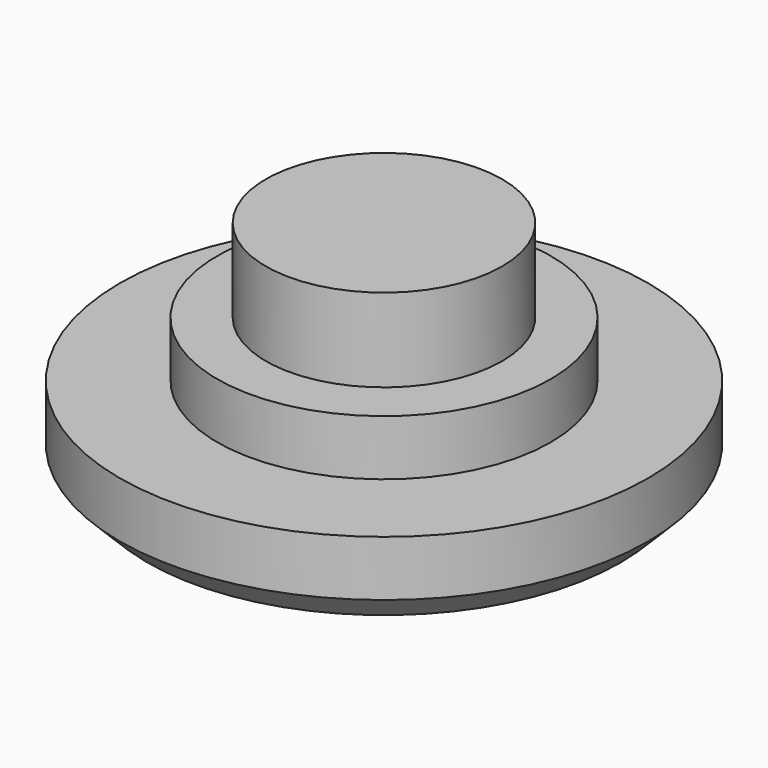
from build123d import *

# Parameters (mm, degrees)
F2_R         = 9.5
F2_R_2       = 6
F3_DEPTH     = 3
F2_R_3       = 4.25
F4_DEPTH     = 5
F5_DEPTH     = 8
F6_SIZE      = 1
F7_TEXT_SIZE = 15.047749256
F8_DEPTH     = 1


# Not quite as in the source:
# - Text() gives the source's letters only with a copy of the font that has no kerning and outlines rounded to 1/6400 em; it was checked with that copy


with BuildPart() as f3:
    # F2 (on Top) → F3 (new body)
    with BuildSketch(Plane.XY):
        Circle(F2_R)
        Circle(F2_R_2, mode=Mode.SUBTRACT)
    extrude(amount=F3_DEPTH)

    # F2 (on Top) → F4 (join)
    with BuildSketch(Plane.XY):
        Circle(F2_R_2)
        Circle(F2_R_3, mode=Mode.SUBTRACT)
    extrude(amount=F4_DEPTH)

    # F2 (on Top) → F5 (join)
    with BuildSketch(Plane.XY):
        Circle(F2_R_3)
    extrude(amount=F5_DEPTH)

    # F6
    f6_edges = [f3.edges().sort_by_distance(p)[0] for p in [
        (-9.5, 0, 0),
    ]]
    chamfer(f6_edges, length=F6_SIZE)

    # F7 (on face) → F8 (cut)
    with BuildSketch(Plane(origin=(0, 0, 0), x_dir=(1, 0, 0), z_dir=(0, 0, -1))):
        with Locations((-6.6979058399, -5.6010194194)):
            Text('M', F7_TEXT_SIZE, font='Open Sans', text_align=(TextAlign.LEFT, TextAlign.BOTTOM))
    extrude(amount=-F8_DEPTH, mode=Mode.SUBTRACT)


solid = f3.part
